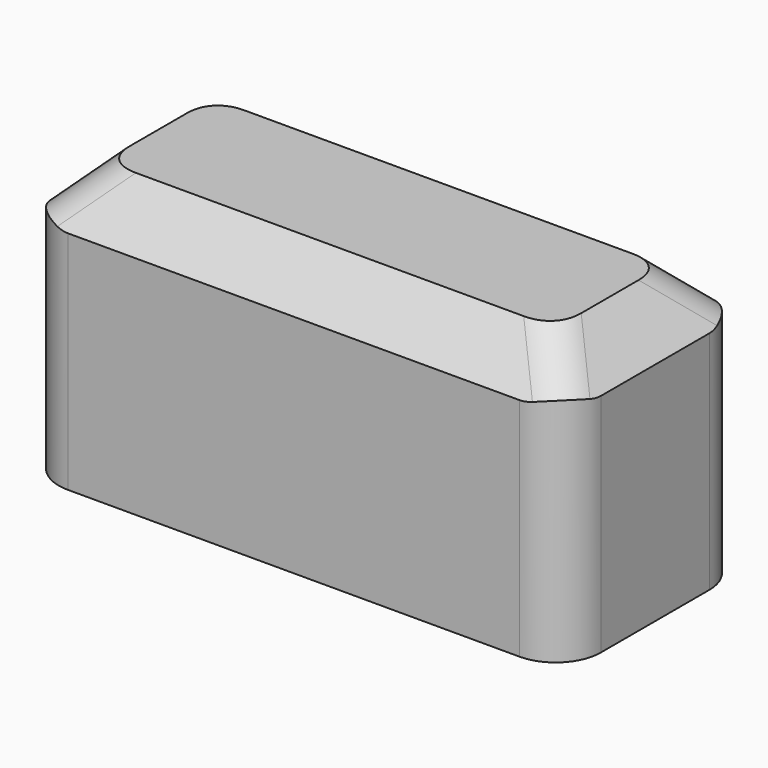
from build123d import *

# Parameters (mm, degrees)
F0_W     = 60
F0_H     = 25
F1_DEPTH = 30
F2_SIZE  = 5
F3_F1_R  = 5
F3_F2_R  = 5
F3_F3_R  = 5
F3_F4_R  = 5
F3_F5_R  = 5
F3_F6_R  = 5
F3_F7_R  = 5
F3_F8_R  = 5
F5_DEPTH = 25


with BuildPart() as f1:
    # F0 (on Top) → F1 (new body)
    with BuildSketch(Plane.XY):
        Rectangle(F0_W, F0_H)
    extrude(amount=F1_DEPTH)

    # F2
    f2_edges = [f1.edges().sort_by_distance(p)[0] for p in [
        (-30, 0, 30),
        (0, -12.5, 30),
        (30, 0, 30),
        (0, 12.5, 30),
    ]]
    chamfer(f2_edges, length=F2_SIZE)

    # F3: fillet of radius 5 on 8 edges, made by hand

    # F3_f1
    f3_f1_edges = [f1.edges().sort_by_distance(p)[0] for p in [
        (-30, 12.5, 12.5),
    ]]
    fillet(f3_f1_edges, radius=F3_F1_R)

    # F3_f2
    f3_f2_edges = [f1.edges().sort_by_distance(p)[0] for p in [
        (-30, -12.5, 12.5),
    ]]
    fillet(f3_f2_edges, radius=F3_F2_R)

    # F3_f3
    f3_f3_edges = [f1.edges().sort_by_distance(p)[0] for p in [
        (30, 12.5, 12.5),
    ]]
    fillet(f3_f3_edges, radius=F3_F3_R)

    # F3_f4
    f3_f4_edges = [f1.edges().sort_by_distance(p)[0] for p in [
        (-26.767766953, 9.267766953, 28.232233047),
    ]]
    fillet(f3_f4_edges, radius=F3_F4_R)

    # F3_f5
    f3_f5_edges = [f1.edges().sort_by_distance(p)[0] for p in [
        (-26.767766953, -9.267766953, 28.232233047),
    ]]
    fillet(f3_f5_edges, radius=F3_F5_R)

    # F3_f6
    f3_f6_edges = [f1.edges().sort_by_distance(p)[0] for p in [
        (30, -12.5, 12.5),
    ]]
    fillet(f3_f6_edges, radius=F3_F6_R)

    # F3_f7
    f3_f7_edges = [f1.edges().sort_by_distance(p)[0] for p in [
        (26.767766953, 9.267766953, 28.232233047),
    ]]
    fillet(f3_f7_edges, radius=F3_F7_R)

    # F3_f8
    f3_f8_edges = [f1.edges().sort_by_distance(p)[0] for p in [
        (26.767766953, -9.267766953, 28.232233047),
    ]]
    fillet(f3_f8_edges, radius=F3_F8_R)

    # F4 (on face) → F5 (cut)
    with BuildSketch(Plane(origin=(0, 0, 0), x_dir=(1, 0, 0), z_dir=(0, 0, -1))):
        with BuildLine():
            ThreePointArc((-25, -2.5), (-23.5355339059, -6.0355339059), (-20, -7.5))
            Line((-20, -7.5), (20, -7.5))
            ThreePointArc((20, -7.5), (23.5355339059, -6.0355339059), (25, -2.5))
            Line((25, -2.5), (25, 2.5))
            ThreePointArc((25, 2.5), (23.5355339059, 6.0355339059), (20, 7.5))
            Line((20, 7.5), (-20, 7.5))
            ThreePointArc((-20, 7.5), (-23.5355339059, 6.0355339059), (-25, 2.5))
            Line((-25, 2.5), (-25, -2.5))
        make_face()
    extrude(amount=-F5_DEPTH, mode=Mode.SUBTRACT)


solid = f1.part
